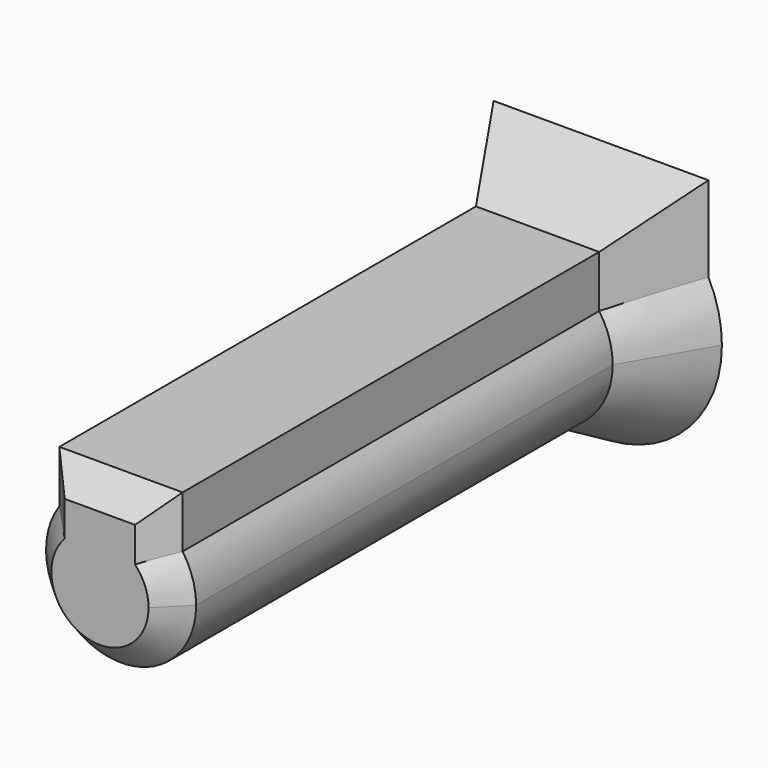
from build123d import *

# Parameters (mm, degrees)
F1_DEPTH               = 103.5
F2_DEPTH               = 15
DRAFT_F2_DRAFTED_ANGLE = -30
F3_SIZE                = 5


# Not quite as in the source:
# - an extrude with a draft is written as a straight extrude whose walls are then drafted


with BuildPart() as f1:
    # F0 (on Front) → F1 (new body)
    with BuildSketch(Plane.XZ):
        with BuildLine():
            ThreePointArc((-11.6774164984, 8.0664324248), (-4.2247304745, -13.5492081155), (14.1925821519, 0))
            ThreePointArc((14.1925821519, 0), (13.5394209568, 4.2559920459), (11.6400560364, 8.1202514498))
            ThreePointArc((11.6400560364, 8.1202514498), (-0.0327577913, 14.1925443479), (-11.6774164984, 8.0664324248))
        make_face()
        with BuildLine():
            ThreePointArc((-11.6774164984, 8.0664324248), (-0.0327577913, 14.1925443479), (11.6400560364, 8.1202514498))
            Line((11.6400560364, 8.1202514498), (11.6400560364, 17.9630486791))
            Line((11.6400560364, 17.9630486791), (-11.6774164984, 17.9630486791))
            Line((-11.6774164984, 17.9630486791), (-11.6774164984, 8.0664324248))
        make_face()
    extrude(amount=F1_DEPTH)


with BuildPart() as f2_drafted:
    # F2 (new): a face of the model
    f2_faces = [f1.part.faces().sort_by_distance(p)[0] for p in [
        (-0.0056333684, 0, 2.5444837056),
    ]]
    extrude(f2_faces, amount=F2_DEPTH)

    # draft_F2_drafted
    draft_f2_drafted_walls = [f2_drafted.faces().sort_by_distance(p)[0] for p in [
        (0.0327577913, 10, -14.1925443479),
        (11.6400560364, 10, 13.0416500645),
        (-0.018680231, 10, 17.9630486791),
        (-11.6774164984, 10, 13.014740552),
    ]]
    draft(draft_f2_drafted_walls, neutral_plane=Plane(origin=(-0.0056333684, 0, 2.5444837056), x_dir=(1, 0, 0), z_dir=(0, 1, 0)), angle=DRAFT_F2_DRAFTED_ANGLE)


with BuildPart() as f1_1:
    add(f1.part)

    # join_F2_drafted: union F2_drafted
    add(f2_drafted.part)

    # F3
    f3_edges = [f1_1.edges().sort_by_distance(p)[0] for p in [
        (0.032758, -103.5, -14.192544),
        (11.640056, -103.5, 13.04165),
        (-0.01868, -103.5, 17.963049),
        (-11.677416, -103.5, 13.014741),
    ]]
    chamfer(f3_edges, length=F3_SIZE)


solid = f1_1.part
